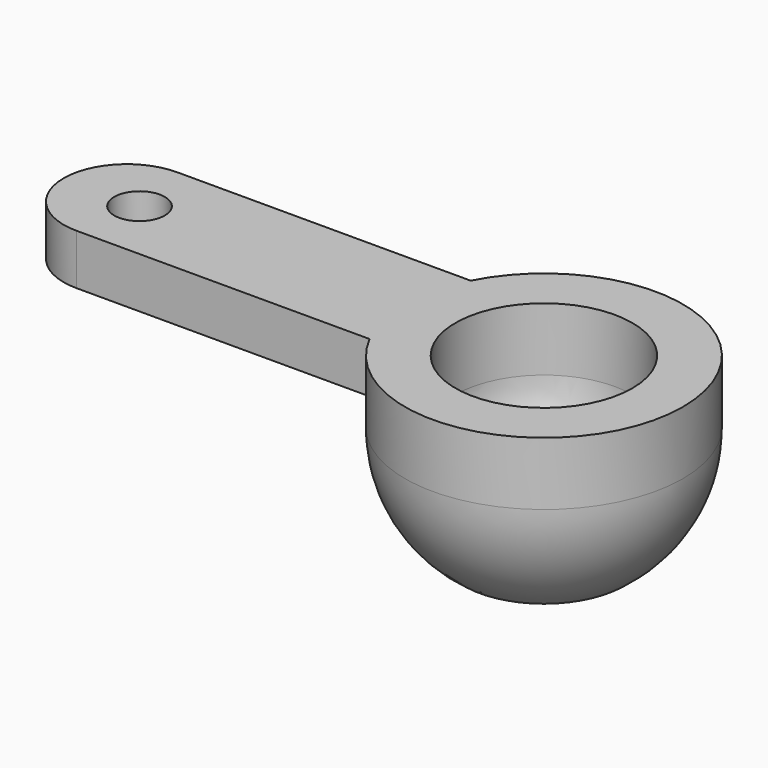
from build123d import *

# Parameters (mm, degrees)
F0_W      = 19
F0_H      = 5
F1_DEPTH  = 2
F4_ANGLE  = 180
F5_R      = 5.5
F6_DEPTH  = 2.5
F7_R      = 3.5
F8_DEPTH  = 2.5
F11_W     = 20
F11_H     = 5
F12_DEPTH = 12.5
F13_W     = 5
F13_H     = 2.5
F14_DEPTH = 25
F15_R     = 1
F16_DEPTH = 25
F17_R     = 2.49999


# Not quite as in the source:
# - a fillet or chamfer is up to 0.001 mm smaller than in the source, because OpenCascade refuses the exact size


with BuildPart() as f1:
    # F0 (on Top) → F1 (new body)
    with BuildSketch(Plane.XY):
        with Locations((6.5, 0)):
            Rectangle(F0_W, F0_H)
    extrude(amount=F1_DEPTH)



with BuildPart() as f4:
    # F3 (on offset) → F4 (revolve)
    with BuildSketch(Plane.XY.offset(-0.5)):
        with BuildLine():
            ThreePointArc((21.5, 0), (16, 5.5), (10.5, 0))
            Line((10.5, 0), (21.5, 0))
        make_face()
    revolve(axis=Axis((22.6478228122, 0, -0.5), (-1, 0, 0)), revolution_arc=F4_ANGLE)


with BuildPart() as f1_1:
    add(f1.part)

    add(f4.part)  # F6 merges F4
    # F5 (on offset) → F6 (join, through all)
    with BuildSketch(Plane.XY.offset(-0.5)):
        with Locations((16, 0)):
            Circle(F5_R)
    extrude(amount=F6_DEPTH)

    # F7 (on offset) → F8 (cut, through all)
    with BuildSketch(Plane.XY.offset(-0.5)):
        with Locations((16, 0)):
            Circle(F7_R)
    extrude(amount=F8_DEPTH, mode=Mode.SUBTRACT)

    # F9 (on offset) → F10 (revolve, cut)
    with BuildSketch(Plane.XY.offset(-0.5)):
        with BuildLine():
            ThreePointArc((12.5, 0), (16, -3.5), (19.5, 0))
            Line((19.5, 0), (12.5, 0))
        make_face()
    revolve(axis=Axis((18.6947258189, 0, -0.5), (1, 0, 0)), mode=Mode.SUBTRACT)

    # F11 (on Front) → F12 (cut, symmetric)
    with BuildSketch(Plane.XZ):
        with Locations((16, -7.5)):
            Rectangle(F11_W, F11_H)
    extrude(amount=F12_DEPTH, both=True, mode=Mode.SUBTRACT)

    # F13 (on Top) → F14 (cut)
    with BuildSketch(Plane.XY):
        with Locations((16, 0)):
            Rectangle(F13_W, F13_H)
    extrude(amount=-F14_DEPTH, mode=Mode.SUBTRACT)

    # F15 (on Top) → F16 (cut)
    with BuildSketch(Plane.XY):
        Circle(F15_R)
    extrude(amount=F16_DEPTH, mode=Mode.SUBTRACT)

    # F17 (radius 2.5 in the source; OpenCascade refuses exactly that, so slightly less here)
    f17_edges = [f1_1.edges().sort_by_distance(p)[0] for p in [
        (-3, -2.5, 1),
        (-3, 2.5, 1),
    ]]
    fillet(f17_edges, radius=F17_R)


solid = f1_1.part
